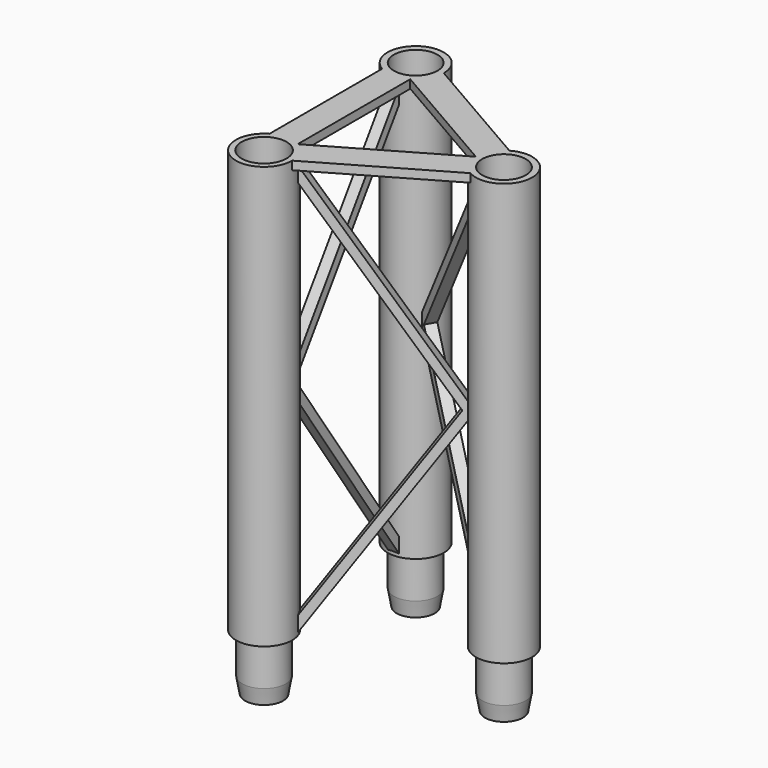
from build123d import *

# Parameters (mm, degrees)
F1_DEPTH  = 3
F2_R      = 10
F3_DEPTH  = 150
F4_W      = 4
F4_H      = 47.7245901334
F5_DEPTH  = 146
F7_DEPTH  = 146
F9_DEPTH  = 146
F11_DEPTH = 4
F13_DEPTH = 4
F15_DEPTH = 4
F16_R     = 10
F17_DEPTH = 150
F18_R     = 8
F19_DEPTH = 135
F20_R     = 7.75
F21_DEPTH = 20
F22_SIZE2 = 5.6712818196
F22_SIZE  = 1
F23_R     = 5
F24_DEPTH = 30
F25_R     = 7.75
F26_DEPTH = 20
F27_SIZE2 = 5.6712818196
F27_SIZE  = 1
F28_R     = 5
F29_DEPTH = 30
F30_R     = 7.75
F31_DEPTH = 20
F32_SIZE2 = 5.6712818196
F32_SIZE  = 1
F33_R     = 5
F34_DEPTH = 30
F35_R     = 10
F35_R_2   = 7.75
F36_DEPTH = 150
F37_R     = 10
F37_R_2   = 7.75
F38_DEPTH = 150


# Not quite as in the source:
# - a feature names something its author has since deleted; it is built from what else it names


with BuildPart() as f1:
    # F0 (on Top) → F1 (new body)
    with BuildSketch(Plane.XY):
        Polygon((63.3012701892, -25), (-10, 17.3205080757), (-10, -67.3205080757), align=None)
        Polygon((0, -50), (0, 0), (43.3012701892, -25), align=None, mode=Mode.SUBTRACT)
    extrude(amount=F1_DEPTH)

    # F2 (on face) → F3 (join)
    with BuildSketch(Plane.XY.offset(3)):
        with Locations((-5, 8.6602540378)):
            Circle(F2_R)
        with Locations((53.3012701892, -25)):
            Circle(F2_R)
        with Locations((-5, -58.6602540378)):
            Circle(F2_R)
    extrude(amount=-F3_DEPTH)

    # F4 (on face) → F5 (join)
    with BuildSketch(Plane(origin=(0, 0, 0), x_dir=(1, 0, 0), z_dir=(0, 0, -1))):
        with Locations((-5, 25)):
            Rectangle(F4_W, F4_H)
    extrude(amount=F5_DEPTH)

    # F6 (on face) → F7 (join)
    with BuildSketch(Plane(origin=(0, 0, 0), x_dir=(1, 0, 0), z_dir=(0, 0, -1))):
        Polygon((4.4852813742, -5.4933253598), (45.815988815, 18.3689697069), (43.815988815, 21.833071322), (2.4852813742, -2.0292237447), align=None)
    extrude(amount=F7_DEPTH)

    # F8 (on face) → F9 (join)
    with BuildSketch(Plane(origin=(0, 0, 0), x_dir=(1, 0, 0), z_dir=(0, 0, -1))):
        Polygon((43.815988815, 28.166928678), (45.815988815, 31.6310302931), (4.4852813742, 55.4933253598), (2.4852813742, 52.0292237447), align=None)
    extrude(amount=F9_DEPTH)

    # F10 (on face) → F11 (cut, through all)
    with BuildSketch(Plane(origin=(-7, 0, 0), x_dir=(0, -1, 0), z_dir=(-1, 0, 0))):
        Polygon((48.8622950667, -76), (1.1377049333, -146), (48.8622950667, -146), align=None)
        Polygon((48.8622950667, -70), (48.8622950667, 0), (1.1377049333, 0), align=None)
        Polygon((1.1377049333, -5.3256151295), (1.1377049333, -140.6743848705), (47.2767375115, -73), align=None)
    extrude(amount=-F11_DEPTH, mode=Mode.SUBTRACT)

    # F12 (on face) → F13 (cut, through all)
    with BuildSketch(Plane(origin=(3.5, 6.0621778265, 0), x_dir=(-0.8660254038, 0.5, 0), z_dir=(0.5, 0.8660254038, 0))):
        Polygon((-1.1377049333, -76), (-48.8622950667, -146), (-1.1377049333, -146), align=None)
        Polygon((-1.1377049333, -70), (-1.1377049333, 0), (-48.8622950667, 0), align=None)
        Polygon((-48.8622950667, -5.3256151295), (-48.8622950667, -140.6743848705), (-2.7232624885, -73), align=None)
    extrude(amount=-F13_DEPTH, mode=Mode.SUBTRACT)

    # F14 (on face) → F15 (cut, through all)
    with BuildSketch(Plane(origin=(25.1506350946, -43.5621778265, 0), x_dir=(0.8660254038, 0.5, 0), z_dir=(0.5, -0.8660254038, 0))):
        Polygon((23.8622950667, -76), (-23.8622950667, -146), (23.8622950667, -146), align=None)
        Polygon((23.8622950667, -70), (23.8622950667, 0), (-23.8622950667, 0), align=None)
        Polygon((-23.8622950667, -5.3256151295), (-23.8622950667, -140.6743848705), (22.2767375115, -73), align=None)
    extrude(amount=-F15_DEPTH, mode=Mode.SUBTRACT)

    # F16 (on face) → F17 (join)
    with BuildSketch(Plane(origin=(0, 0, -147), x_dir=(1, 0, 0), z_dir=(0, 0, -1))):
        with Locations((-5, 58.6602540378)):
            Circle(F16_R)
    extrude(amount=-F17_DEPTH)

    # F18 (on face) → F19 (cut)
    with BuildSketch(Plane.XY.offset(3)):
        with Locations((-5, 8.6602540378)):
            Circle(F18_R)
        with Locations((53.3012701892, -25)):
            Circle(F18_R)
        with Locations((-5, -58.6602540378)):
            Circle(F18_R)
    extrude(amount=-F19_DEPTH, mode=Mode.SUBTRACT)

    # F20 (on face) → F21 (join)
    with BuildSketch(Plane(origin=(0, 0, -147), x_dir=(1, 0, 0), z_dir=(0, 0, -1))):
        with Locations((-5, 58.6602540378)):
            Circle(F20_R)
    extrude(amount=F21_DEPTH)

    # F22
    f22_edges = [f1.edges().sort_by_distance(p)[0] for p in [
        (-12.75, -58.660254, -167),
    ]]
    f22_side = f1.faces().sort_by_distance((-5, -58.660254, -167))[0]
    chamfer(f22_edges, length=F22_SIZE, length2=F22_SIZE2, reference=f22_side)

    # F23 (on face) → F24 (cut)
    with BuildSketch(Plane.XY.offset(-132)):
        with Locations((-5, -58.6602540378)):
            Circle(F23_R)
    extrude(amount=-F24_DEPTH, mode=Mode.SUBTRACT)

    # F25 (on face) → F26 (join)
    with BuildSketch(Plane(origin=(0, 0, -147), x_dir=(1, 0, 0), z_dir=(0, 0, -1))):
        with Locations((53.3012701892, 25)):
            Circle(F25_R)
    extrude(amount=F26_DEPTH)

    # F27
    f27_edges = [f1.edges().sort_by_distance(p)[0] for p in [
        (45.55127, -25, -167),
    ]]
    f27_side = f1.faces().sort_by_distance((53.30127, -25, -167))[0]
    chamfer(f27_edges, length=F27_SIZE, length2=F27_SIZE2, reference=f27_side)

    # F28 (on face) → F29 (cut)
    with BuildSketch(Plane.XY.offset(-132)):
        with Locations((53.3012701892, -25)):
            Circle(F28_R)
    extrude(amount=-F29_DEPTH, mode=Mode.SUBTRACT)

    # F30 (on face) → F31 (join)
    with BuildSketch(Plane(origin=(0, 0, -147), x_dir=(1, 0, 0), z_dir=(0, 0, -1))):
        with Locations((-5, -8.6602540378)):
            Circle(F30_R)
    extrude(amount=F31_DEPTH)

    # F32
    f32_edges = [f1.edges().sort_by_distance(p)[0] for p in [
        (-12.75, 8.660254, -167),
    ]]
    f32_side = f1.faces().sort_by_distance((-5, 8.660254, -167))[0]
    chamfer(f32_edges, length=F32_SIZE, length2=F32_SIZE2, reference=f32_side)

    # F33 (on face) → F34 (cut)
    with BuildSketch(Plane.XY.offset(-132)):
        with Locations((-5, 8.6602540378)):
            Circle(F33_R)
    extrude(amount=-F34_DEPTH, mode=Mode.SUBTRACT)

    # F35 (on face) → F36 (join)
    with BuildSketch(Plane(origin=(0, 0, -147), x_dir=(1, 0, 0), z_dir=(0, 0, -1))):
        with Locations((-5, -8.6602540378)):
            Circle(F35_R)
        with Locations((-5, -8.6602540378)):
            Circle(F35_R_2, mode=Mode.SUBTRACT)
    extrude(amount=-F36_DEPTH)

    # F37 (on face) → F38 (join)
    with BuildSketch(Plane(origin=(0, 0, -147), x_dir=(1, 0, 0), z_dir=(0, 0, -1))):
        with Locations((53.3012701892, 25)):
            Circle(F37_R)
        with Locations((53.3012701892, 25)):
            Circle(F37_R_2, mode=Mode.SUBTRACT)
    extrude(amount=-F38_DEPTH)


solid = f1.part
